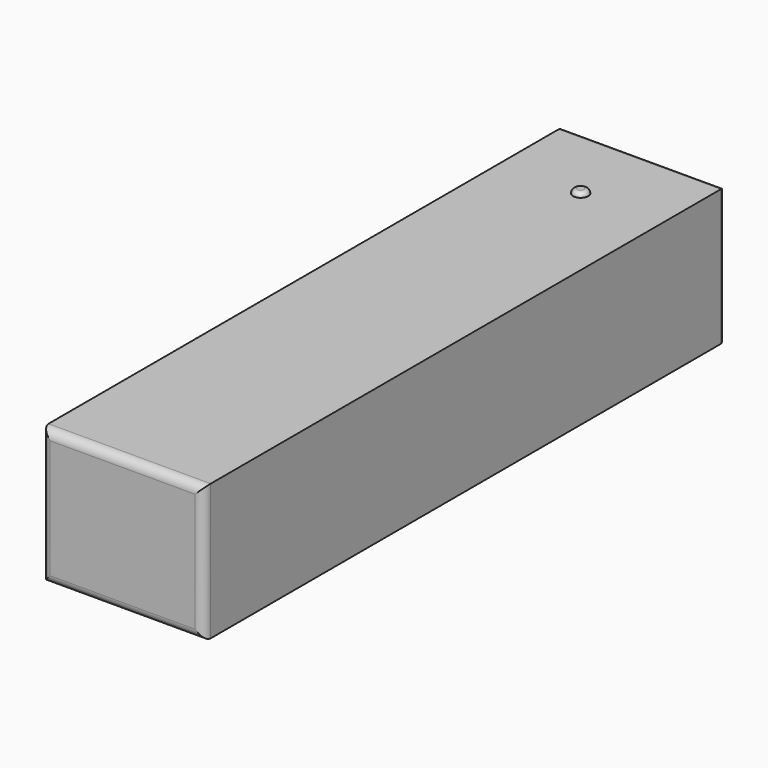
from build123d import *

# Parameters (mm, degrees)
F0_W      = 37.4
F0_H      = 31.4
F0_W_2    = 15.7
F0_H_2    = 2.9
F1_DEPTH  = 147
F2_W      = 37.4
F2_H      = 31.4
F3_DEPTH  = 3
F4_R      = 2
F5_R      = 0.99999
F7_R      = 1.75
F8_DEPTH  = 1
F9_R      = 0.99999
F11_R     = 1.75
F12_DEPTH = 1
F13_R     = 0.99999


# Not quite as in the source:
# - a fillet or chamfer is up to 0.001 mm smaller than in the source, because OpenCascade refuses the exact size


with BuildPart() as f1:
    # F0 (on Front) → F1 (new body)
    with BuildSketch(Plane.XZ):
        with Locations((1, -17.2441455504)):
            Rectangle(F0_W, F0_H)
        with Locations((-7.85, -29.4941455504)):
            Rectangle(F0_W_2, F0_H_2, mode=Mode.SUBTRACT)
        with Locations((-7.85, -24.5941455504)):
            Rectangle(F0_W_2, F0_H_2, mode=Mode.SUBTRACT)
        with Locations((-7.85, -19.6941455504)):
            Rectangle(F0_W_2, F0_H_2, mode=Mode.SUBTRACT)
        with Locations((9.85, -29.4941455504)):
            Rectangle(F0_W_2, F0_H_2, mode=Mode.SUBTRACT)
        with Locations((9.85, -24.5941455504)):
            Rectangle(F0_W_2, F0_H_2, mode=Mode.SUBTRACT)
        with Locations((9.85, -19.6941455504)):
            Rectangle(F0_W_2, F0_H_2, mode=Mode.SUBTRACT)
        with Locations((-7.85, -14.7941455504)):
            Rectangle(F0_W_2, F0_H_2, mode=Mode.SUBTRACT)
        with Locations((-7.85, -9.8941455504)):
            Rectangle(F0_W_2, F0_H_2, mode=Mode.SUBTRACT)
        with Locations((-7.85, -4.9941455504)):
            Rectangle(F0_W_2, F0_H_2, mode=Mode.SUBTRACT)
        with Locations((9.85, -14.7941455504)):
            Rectangle(F0_W_2, F0_H_2, mode=Mode.SUBTRACT)
        with Locations((9.85, -9.8941455504)):
            Rectangle(F0_W_2, F0_H_2, mode=Mode.SUBTRACT)
        with Locations((9.85, -4.9941455504)):
            Rectangle(F0_W_2, F0_H_2, mode=Mode.SUBTRACT)
    extrude(amount=F1_DEPTH)

    # F2 (on face) → F3 (join)
    with BuildSketch(Plane.XZ.offset(147)):
        with Locations((1, -17.2441455504)):
            Rectangle(F2_W, F2_H)
    extrude(amount=F3_DEPTH)

    # F4
    f4_edges = [f1.edges().sort_by_distance(p)[0] for p in [
        (1, -150, -1.544146),
        (-17.7, -150, -17.244146),
        (1, -150, -32.944146),
        (19.7, -150, -17.244146),
    ]]
    fillet(f4_edges, radius=F4_R)

    # F5 (radius 1 in the source; OpenCascade refuses exactly that, so slightly less here)
    f5_edges = [f1.edges().sort_by_distance(p)[0] for p in [
        (1, 0, -1.544146),
        (-17.7, 0, -17.244146),
        (1, 0, -32.944146),
        (19.7, 0, -17.244146),
        (-15.7, 0, -29.494146),
        (-7.85, 0, -28.044146),
        (0, 0, -29.494146),
        (-7.85, 0, -30.944146),
        (-15.7, 0, -24.594146),
        (-7.85, 0, -23.144146),
        (0, 0, -24.594146),
        (-7.85, 0, -26.044146),
        (-15.7, 0, -19.694146),
        (-7.85, 0, -18.244146),
        (0, 0, -19.694146),
        (-7.85, 0, -21.144146),
        (2, 0, -29.494146),
        (9.85, 0, -28.044146),
        (17.7, 0, -29.494146),
        (9.85, 0, -30.944146),
        (2, 0, -24.594146),
        (9.85, 0, -23.144146),
        (17.7, 0, -24.594146),
        (9.85, 0, -26.044146),
        (2, 0, -19.694146),
        (9.85, 0, -18.244146),
        (17.7, 0, -19.694146),
        (9.85, 0, -21.144146),
        (-15.7, 0, -14.794146),
        (-7.85, 0, -13.344146),
        (0, 0, -14.794146),
        (-7.85, 0, -16.244146),
        (-15.7, 0, -9.894146),
        (-7.85, 0, -8.444146),
        (0, 0, -9.894146),
        (-7.85, 0, -11.344146),
        (-15.7, 0, -4.994146),
        (-7.85, 0, -3.544146),
        (0, 0, -4.994146),
        (-7.85, 0, -6.444146),
        (2, 0, -14.794146),
        (9.85, 0, -13.344146),
        (17.7, 0, -14.794146),
        (9.85, 0, -16.244146),
        (2, 0, -9.894146),
        (9.85, 0, -8.444146),
        (17.7, 0, -9.894146),
        (9.85, 0, -11.344146),
        (2, 0, -4.994146),
        (9.85, 0, -3.544146),
        (17.7, 0, -4.994146),
        (9.85, 0, -6.444146),
    ]]
    fillet(f5_edges, radius=F5_R)

    # F7 (on face) → F8 (join)
    with BuildSketch(Plane.XY.offset(-1.5441455504)):
        with Locations((1, -18)):
            Circle(F7_R)
    extrude(amount=F8_DEPTH)

    # F9 (radius 1 in the source; OpenCascade refuses exactly that, so slightly less here)
    f9_edges = [f1.edges().sort_by_distance(p)[0] for p in [
        (-0.75, -18, -0.544146),
    ]]
    fillet(f9_edges, radius=F9_R)

    # F11 (on face) → F12 (join)
    with BuildSketch(Plane(origin=(0, 0, -32.9441455504), x_dir=(1, 0, 0), z_dir=(0, 0, -1))):
        with Locations((1, 18)):
            Circle(F11_R)
    extrude(amount=F12_DEPTH)

    # F13 (radius 1 in the source; OpenCascade refuses exactly that, so slightly less here)
    f13_edges = [f1.edges().sort_by_distance(p)[0] for p in [
        (-0.75, -18, -33.944146),
    ]]
    fillet(f13_edges, radius=F13_R)


solid = f1.part
